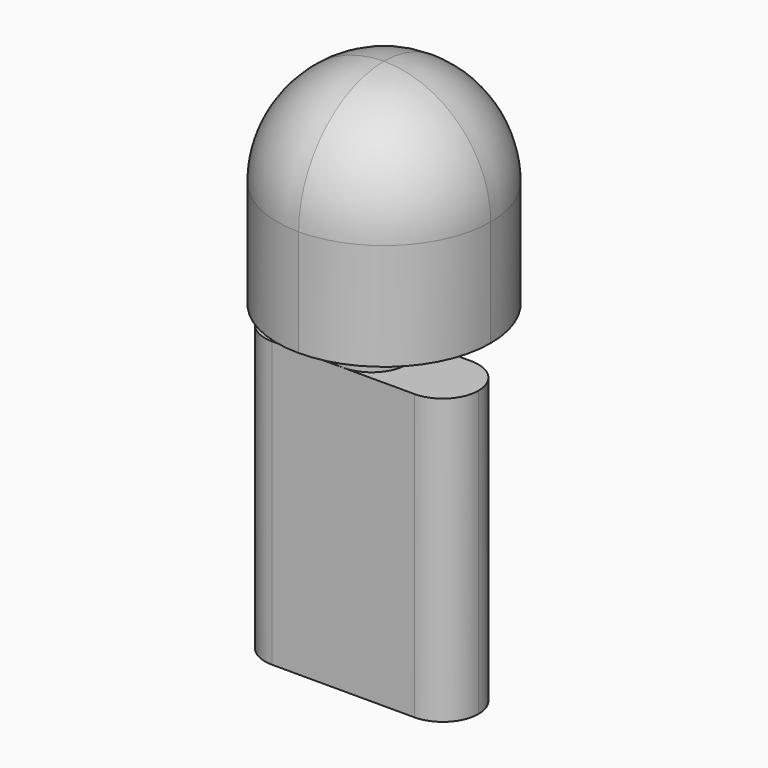
from build123d import *

# Parameters (mm, degrees)
F0_W     = 10
F0_H     = 40
F1_DEPTH = 30
F2_R     = 4.99999
F3_R     = 5
F4_DEPTH = 5
F5_W     = 30
F5_H     = 30
F6_DEPTH = 30
F7_R     = 14.99999


# Not quite as in the source:
# - a fillet or chamfer is up to 0.001 mm smaller than in the source, because OpenCascade refuses the exact size


with BuildPart() as f1:
    # F0 (on Right) → F1 (new body)
    with BuildSketch(Plane.YZ):
        with Locations((5, 20)):
            Rectangle(F0_W, F0_H)
    extrude(amount=-F1_DEPTH)

    # F2 (radius 5 in the source; OpenCascade refuses exactly that, so slightly less here)
    f2_edges = [f1.edges().sort_by_distance(p)[0] for p in [
        (0, 10, 20),
        (0, 0, 20),
        (-30, 10, 20),
        (-30, 0, 20),
    ]]
    fillet(f2_edges, radius=F2_R)

    # F3 (on face) → F4 (join)
    with BuildSketch(Plane.XY.offset(40)):
        with Locations((-15, 5)):
            Circle(F3_R)
    extrude(amount=F4_DEPTH)

    # F5 (on face) → F6 (join)
    with BuildSketch(Plane.XY.offset(45)):
        with Locations((-15, 7.1624371922)):
            Rectangle(F5_W, F5_H)
    extrude(amount=F6_DEPTH)

    # F7 (radius 15 in the source; OpenCascade refuses exactly that, so slightly less here)
    f7_edges = [f1.edges().sort_by_distance(p)[0] for p in [
        (-15, -7.837563, 75),
        (0, 7.162437, 75),
        (-15, 22.162437, 75),
        (-30, 7.162437, 75),
        (-30, 22.162437, 60),
        (0, 22.162437, 60),
        (0, -7.837563, 60),
        (-30, -7.837563, 60),
    ]]
    fillet(f7_edges, radius=F7_R)


solid = f1.part
